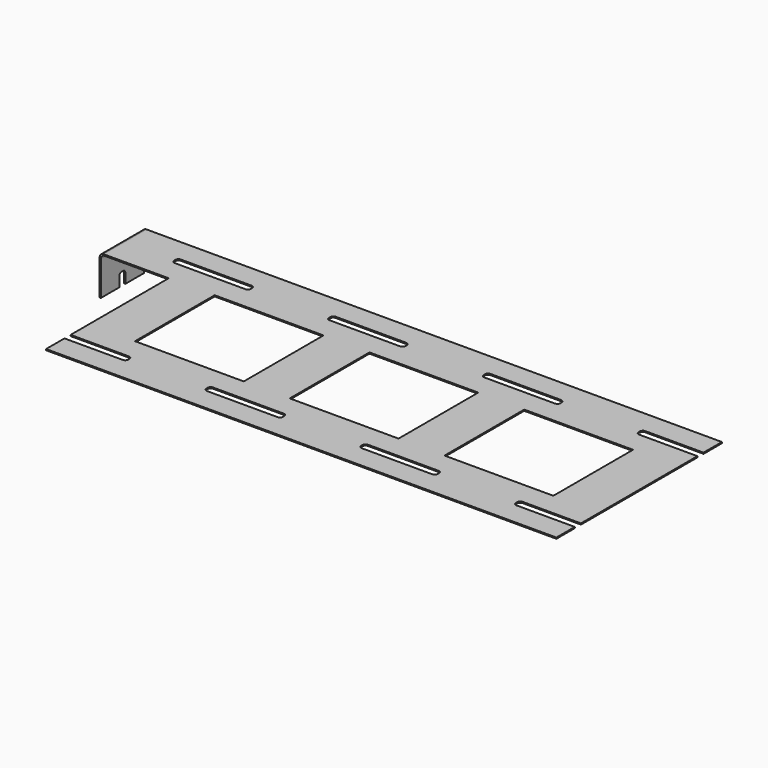
from build123d import *

# Parameters (mm, degrees)
F0_W     = 14.2
F0_H     = 13
F1_DEPTH = 0.15
F2_W     = 0.15
F2_H     = 7
F3_DEPTH = 5
F4_R     = 0.5
F6_DEPTH = 25


# Not quite as in the source:
# - a feature names something its author has since deleted; it is built from what else it names


with BuildPart() as f1:
    # F0 (on Top) → F1 (new body)
    with BuildSketch(Plane.XY):
        with BuildLine():
            Line((-13.1, 10.5), (-13.1, 13.5))
            Line((-13.1, 13.5), (-22.1, 13.5))
            Line((-22.1, 13.5), (-22.1, 6.5))
            Line((-22.1, 6.5), (-13.1, 6.5))
            Line((-13.1, 6.5), (-13.1, 9.5))
            Line((-13.1, 9.5), (-14.7, 9.5))
            ThreePointArc((-14.7, 9.5), (-14.9828427125, 9.6171572875), (-15.1, 9.9))
            Line((-15.1, 9.9), (-15.1, 10.1))
            ThreePointArc((-15.1, 10.1), (-14.9828427125, 10.3828427125), (-14.7, 10.5))
            Line((-14.7, 10.5), (-13.1, 10.5))
        make_face()
        with BuildLine():
            Line((13.1, 10.5), (13.1, 13.5))
            Line((13.1, 13.5), (-7.1, 13.5))
            Line((-7.1, 13.5), (-13.1, 13.5))
            Line((-13.1, 13.5), (-13.1, 10.5))
            Line((-13.1, 10.5), (-5.5, 10.5))
            ThreePointArc((-5.5, 10.5), (-5.2171572875, 10.3828427125), (-5.1, 10.1))
            Line((-5.1, 10.1), (-5.1, 9.9))
            ThreePointArc((-5.1, 9.9), (-5.2171572875, 9.6171572875), (-5.5, 9.5))
            Line((-5.5, 9.5), (-13.1, 9.5))
            Line((-13.1, 9.5), (-13.1, 6.5))
            Line((-13.1, 6.5), (-13.1, 0))
            Line((-13.1, 0), (-13.1, -6.5))
            Line((-13.1, -6.5), (-13.1, -9.5))
            Line((-13.1, -9.5), (-5.5, -9.5))
            ThreePointArc((-5.5, -9.5), (-5.2171572875, -9.6171572875), (-5.1, -9.9))
            Line((-5.1, -9.9), (-5.1, -10.1))
            ThreePointArc((-5.1, -10.1), (-5.2171572875, -10.3828427125), (-5.5, -10.5))
            Line((-5.5, -10.5), (-13.1, -10.5))
            Line((-13.1, -10.5), (-13.1, -13.5))
            Line((-13.1, -13.5), (-7.1, -13.5))
            Line((-7.1, -13.5), (13.1, -13.5))
            Line((13.1, -13.5), (13.1, -10.5))
            Line((13.1, -10.5), (5.5, -10.5))
            ThreePointArc((5.5, -10.5), (5.2171572875, -10.3828427125), (5.1, -10.1))
            Line((5.1, -10.1), (5.1, -9.9))
            ThreePointArc((5.1, -9.9), (5.2171572875, -9.6171572875), (5.5, -9.5))
            Line((5.5, -9.5), (13.1, -9.5))
            Line((13.1, -9.5), (13.1, -6.5))
            Line((13.1, -6.5), (13.1, 0))
            Line((13.1, 0), (13.1, 6.5))
            Line((13.1, 6.5), (13.1, 9.5))
            Line((13.1, 9.5), (5.5, 9.5))
            ThreePointArc((5.5, 9.5), (5.2171572875, 9.6171572875), (5.1, 9.9))
            Line((5.1, 9.9), (5.1, 10.1))
            ThreePointArc((5.1, 10.1), (5.2171572875, 10.3828427125), (5.5, 10.5))
            Line((5.5, 10.5), (13.1, 10.5))
        make_face()
        Rectangle(F0_W, F0_H, mode=Mode.SUBTRACT)
        with BuildLine():
            Line((33.3, 13.5), (13.1, 13.5))
            Line((13.1, 13.5), (13.1, 10.5))
            Line((13.1, 10.5), (14.7, 10.5))
            ThreePointArc((14.7, 10.5), (14.9828427125, 10.3828427125), (15.1, 10.1))
            Line((15.1, 10.1), (15.1, 9.9))
            ThreePointArc((15.1, 9.9), (14.9828427125, 9.6171572875), (14.7, 9.5))
            Line((14.7, 9.5), (13.1, 9.5))
            Line((13.1, 9.5), (13.1, 6.5))
            Line((13.1, 6.5), (27.3, 6.5))
            Line((27.3, 6.5), (27.3, -6.5))
            Line((27.3, -6.5), (13.1, -6.5))
            Line((13.1, -6.5), (13.1, -9.5))
            Line((13.1, -9.5), (14.7, -9.5))
            ThreePointArc((14.7, -9.5), (14.9828427125, -9.6171572875), (15.1, -9.9))
            Line((15.1, -9.9), (15.1, -10.1))
            ThreePointArc((15.1, -10.1), (14.9828427125, -10.3828427125), (14.7, -10.5))
            Line((14.7, -10.5), (13.1, -10.5))
            Line((13.1, -10.5), (13.1, -13.5))
            Line((13.1, -13.5), (33.3, -13.5))
            Line((33.3, -13.5), (33.3, -10.5))
            Line((33.3, -10.5), (25.7, -10.5))
            ThreePointArc((25.7, -10.5), (25.4171572875, -10.3828427125), (25.3, -10.1))
            Line((25.3, -10.1), (25.3, -9.9))
            ThreePointArc((25.3, -9.9), (25.4171572875, -9.6171572875), (25.7, -9.5))
            Line((25.7, -9.5), (33.3, -9.5))
            Line((33.3, -9.5), (33.3, -6.5))
            Line((33.3, -6.5), (33.3, 0))
            Line((33.3, 0), (33.3, 6.5))
            Line((33.3, 6.5), (33.3, 9.5))
            Line((33.3, 9.5), (25.7, 9.5))
            ThreePointArc((25.7, 9.5), (25.4171572875, 9.6171572875), (25.3, 9.9))
            Line((25.3, 9.9), (25.3, 10.1))
            ThreePointArc((25.3, 10.1), (25.4171572875, 10.3828427125), (25.7, 10.5))
            Line((25.7, 10.5), (33.3, 10.5))
            Line((33.3, 10.5), (33.3, 13.5))
        make_face()
        with BuildLine():
            Line((53.5, 13.5), (33.3, 13.5))
            Line((33.3, 13.5), (33.3, 10.5))
            Line((33.3, 10.5), (34.9, 10.5))
            ThreePointArc((34.9, 10.5), (35.1828427125, 10.3828427125), (35.3, 10.1))
            Line((35.3, 10.1), (35.3, 9.9))
            ThreePointArc((35.3, 9.9), (35.1828427125, 9.6171572875), (34.9, 9.5))
            Line((34.9, 9.5), (33.3, 9.5))
            Line((33.3, 9.5), (33.3, 6.5))
            Line((33.3, 6.5), (47.5, 6.5))
            Line((47.5, 6.5), (47.5, -6.5))
            Line((47.5, -6.5), (33.3, -6.5))
            Line((33.3, -6.5), (33.3, -9.5))
            Line((33.3, -9.5), (34.9, -9.5))
            ThreePointArc((34.9, -9.5), (35.1828427125, -9.6171572875), (35.3, -9.9))
            Line((35.3, -9.9), (35.3, -10.1))
            ThreePointArc((35.3, -10.1), (35.1828427125, -10.3828427125), (34.9, -10.5))
            Line((34.9, -10.5), (33.3, -10.5))
            Line((33.3, -10.5), (33.3, -13.5))
            Line((33.3, -13.5), (53.5, -13.5))
            Line((53.5, -13.5), (53.5, -10.5))
            Line((53.5, -10.5), (45.9, -10.5))
            ThreePointArc((45.9, -10.5), (45.6171572875, -10.3828427125), (45.5, -10.1))
            Line((45.5, -10.1), (45.5, -9.9))
            ThreePointArc((45.5, -9.9), (45.6171572875, -9.6171572875), (45.9, -9.5))
            Line((45.9, -9.5), (53.5, -9.5))
            Line((53.5, -9.5), (53.5, 0))
            Line((53.5, 0), (53.5, 9.5))
            Line((53.5, 9.5), (45.9, 9.5))
            ThreePointArc((45.9, 9.5), (45.6171572875, 9.6171572875), (45.5, 9.9))
            Line((45.5, 9.9), (45.5, 10.1))
            ThreePointArc((45.5, 10.1), (45.6171572875, 10.3828427125), (45.9, 10.5))
            Line((45.9, 10.5), (53.5, 10.5))
            Line((53.5, 10.5), (53.5, 13.5))
        make_face()
    extrude(amount=F1_DEPTH)

    # F2 (on face) → F3 (join)
    with BuildSketch(Plane(origin=(0, 0, 0), x_dir=(1, 0, 0), z_dir=(0, 0, -1))):
        with Locations((-22.025, -10)):
            Rectangle(F2_W, F2_H)
    extrude(amount=F3_DEPTH)

    # F4
    f4_edges = [f1.edges().sort_by_distance(p)[0] for p in [
        (-21.95, 10, 0),
        (-22.1, 10, 0.15),
    ]]
    fillet(f4_edges, radius=F4_R)

    # F5 (on face) → F6 (cut)
    with BuildSketch(Plane(origin=(-22.1, 0, 0), x_dir=(0, -1, 0), z_dir=(-1, 0, 0))):
        with BuildLine():
            Line((-9.9, -3.35), (-10, -3.35))
            Line((-10, -3.35), (-10.1, -3.35))
            ThreePointArc((-10.1, -3.35), (-10.3828427125, -3.4671572875), (-10.5, -3.75))
            Line((-10.5, -3.75), (-10.5, -5))
            Line((-10.5, -5), (-9.5, -5))
            Line((-9.5, -5), (-9.5, -3.75))
            ThreePointArc((-9.5, -3.75), (-9.6171572875, -3.4671572875), (-9.9, -3.35))
        make_face()
    extrude(amount=-F6_DEPTH, mode=Mode.SUBTRACT)


solid = f1.part
